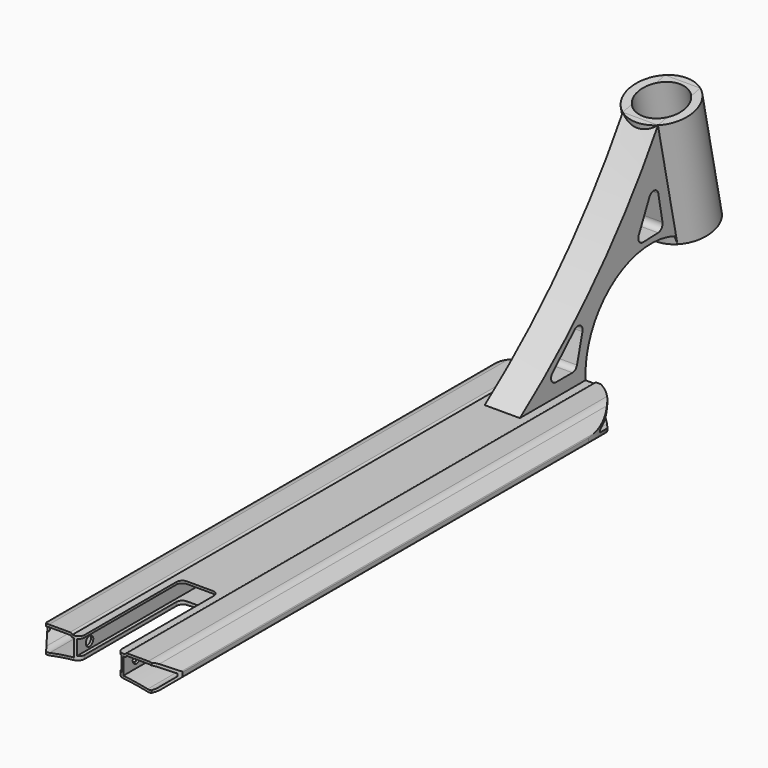
from build123d import *

# Parameters (mm, degrees)
F1_DEPTH       = 250
F2_W           = 38
F2_H           = 13
F3_DEPTH       = 500.001
F4_T1_DEPTH    = 509.3674969976
F5_R           = 9
F6_R           = 1
F8_DEPTH       = 500.001
F10_DEPTH      = 21.9508968951
F10_DEPTH_BACK = 1.301
F12_DEPTH      = 21.9508969951
F12_DEPTH_BACK = 1.3010001
F13_T1_DEPTH   = 2
F13_T6_DEPTH   = 15.5773592081
F13_S7_R       = 200
F13_T8_DEPTH   = 10
F13_T12_DEPTH  = 15.5773592081
F13_S13_R      = 200
F13_T14_DEPTH  = 10
F13_T15_DEPTH  = 28.0773592081
F13_T17_DEPTH  = 27
F15_DEPTH      = 15
F16_R          = 27.5
F17_DEPTH      = 100
F19_D          = 40
F21_D          = 8
F21_DEPTH      = 78.5010001
F23_DEPTH      = 72.5010001
F24_R          = 5


# Not quite as in the source:
# - a fillet or chamfer that OpenCascade refuses, or shapes differently, is made with other operations: its cross-section is extruded or revolved along the edge and cut away or added


with BuildPart() as f1:
    # F0 (on Front) → F1 (new body, symmetric)
    with BuildSketch(Plane.XZ):
        with BuildLine():
            Line((22.5, 0), (0, 0))
            Line((0, 0), (-22.5, 0))
            Line((-22.5, 0), (-22.5, 1.3))
            Line((-22.5, 1.3), (-45.5824640741, 1.3))
            Line((-45.5824640741, 1.3), (-57.5, -8.7))
            Line((-57.5, -8.7), (-57.5, -12.7))
            Line((-57.5, -12.7), (-45.5824640741, -22.7))
            ThreePointArc((-45.5824640741, -22.7), (0, -17.4363319182), (45.5824640741, -22.7))
            Line((45.5824640741, -22.7), (57.5, -12.7))
            Line((57.5, -12.7), (57.5, -8.7))
            Line((57.5, -8.7), (45.5824640741, 1.3))
            Line((45.5824640741, 1.3), (22.5, 1.3))
            Line((22.5, 1.3), (22.5, 0))
        make_face()
    extrude(amount=F1_DEPTH, both=True)

    # F2 (on face) → F3 (cut, through all)
    with BuildSketch(Plane.XZ.offset(250)):
        with Locations((0, -8.5)):
            Rectangle(F2_W, F2_H)
    extrude(amount=-F3_DEPTH, mode=Mode.SUBTRACT)

    # F4: fillet of radius 2 on 2 edges, made by hand

    # F4_s2 → F4_t1 (cut)
    with BuildSketch(Plane.XZ.offset(-254.6837484988)):
        with BuildLine():
            ThreePointArc((-24.3734993995, 1.3), (-23.2333239744, 0.9431676725), (-22.5, 0))
            Line((-22.5, 0), (-22.5, 1.3))
            Line((-22.5, 1.3), (-24.3734993995, 1.3))
        make_face()
        with BuildLine():
            ThreePointArc((24.3734993995, 1.3), (23.2333239744, 0.9431676725), (22.5, 0))
            Line((22.5, 0), (22.5, 1.3))
            Line((22.5, 1.3), (24.3734993995, 1.3))
        make_face()
    extrude(amount=F4_T1_DEPTH, mode=Mode.SUBTRACT)

    # F5
    f5_edges = [f1.edges().sort_by_distance(p)[0] for p in [
        (-45.582464, 0, 1.3),
        (45.582464, 0, 1.3),
        (45.582464, 0, -22.7),
        (-45.582464, 0, -22.7),
    ]]
    fillet(f5_edges, radius=F5_R)

    # F6
    f6_edges = [f1.edges().sort_by_distance(p)[0] for p in [
        (57.5, 0, -8.7),
        (57.5, 0, -12.7),
        (-57.5, 0, -8.7),
        (-57.5, 0, -12.7),
    ]]
    fillet(f6_edges, radius=F6_R)

    # F7 (on face) → F8 (cut, through all)
    with BuildSketch(Plane.XZ.offset(250)):
        with BuildLine():
            ThreePointArc((-41.7537576423, -19.7987248623), (-31.4193924923, -17.8948029689), (-21, -16.5308815192))
            Line((-21, -16.5308815192), (-21, -2))
            Line((-21, -2), (-22.8755325079, -2))
            ThreePointArc((-22.8755325079, -2), (-23.3817957129, -1.070317781), (-24.3734993995, -0.7))
            Line((-24.3734993995, -0.7), (-42.3067319657, -0.7))
            ThreePointArc((-42.3067319657, -0.7), (-44.7008729689, -1.1221516545), (-46.8062452335, -2.3376888982))
            Line((-46.8062452335, -2.3376888982), (-55.5, -9.6326153163))
            Line((-55.5, -9.6326153163), (-55.5, -11.7673846837))
            Line((-55.5, -11.7673846837), (-47.7001833036, -18.3122079969))
            ThreePointArc((-47.7001833036, -18.3122079969), (-44.8983231577, -19.7409184587), (-41.7537576423, -19.7987248623))
        make_face()
        with BuildLine():
            Line((21, -2), (21, -16.5308815192))
            ThreePointArc((21, -16.5308815192), (31.4193924923, -17.8948029689), (41.7537576423, -19.7987248623))
            ThreePointArc((41.7537576423, -19.7987248623), (44.8983231577, -19.7409184587), (47.7001833036, -18.3122079969))
            Line((47.7001833036, -18.3122079969), (55.5, -11.7673846837))
            Line((55.5, -11.7673846837), (55.5, -9.6326153163))
            Line((55.5, -9.6326153163), (46.8062452335, -2.3376888982))
            ThreePointArc((46.8062452335, -2.3376888982), (44.7008729689, -1.1221516545), (42.3067319657, -0.7))
            Line((42.3067319657, -0.7), (24.3734993995, -0.7))
            ThreePointArc((24.3734993995, -0.7), (23.3817957129, -1.070317781), (22.8755325079, -2))
            Line((22.8755325079, -2), (21, -2))
        make_face()
    extrude(amount=-F8_DEPTH, mode=Mode.SUBTRACT)

    # F9 (on Top) → F10 (cut, two sides)
    with BuildSketch(Plane.XY) as f10_sk:
        with BuildLine():
            ThreePointArc((-57.5, 200), (0, 257.5), (57.5, 200))
            Line((57.5, 200), (57.5, 280))
            Line((57.5, 280), (-57.5, 280))
            Line((-57.5, 280), (-57.5, 200))
        make_face()
    extrude(amount=-F10_DEPTH, mode=Mode.SUBTRACT)
    extrude(f10_sk.sketch, amount=F10_DEPTH_BACK, mode=Mode.SUBTRACT)

    # F11 (on Top) → F12 (cut, two sides)
    with BuildSketch(Plane.XY) as f12_sk:
        Polygon((-16, -142.1357727465), (-16, -252.1357727465), (-43.2975540478, -252.1357727465), (-68, -218.1357727465), (-68, -325.6394559335), (0, -325.6394559335), (0, -142.1357727465), align=None)
        Polygon((16, -142.1357727465), (0, -142.1357727465), (0, -325.6394559335), (68, -325.6394559335), (68, -218.1357727465), (43.2975540478, -252.1357727465), (16, -252.1357727465), align=None)
    extrude(amount=-F12_DEPTH, mode=Mode.SUBTRACT)
    extrude(f12_sk.sketch, amount=F12_DEPTH_BACK, mode=Mode.SUBTRACT)

    # F13: fillet of radius 5 on 8 edges, made by hand

    # F13_s2 → F13_t1 (join)
    with BuildSketch(Plane.XY.offset(-2)):
        with BuildLine():
            ThreePointArc((16, -147.1357727465), (14.5355339059, -143.6002388406), (11, -142.1357727465))
            Line((11, -142.1357727465), (16, -142.1357727465))
            Line((16, -142.1357727465), (16, -147.1357727465))
        make_face()
        with BuildLine():
            ThreePointArc((-16, -147.1357727465), (-14.5355339059, -143.6002388406), (-11, -142.1357727465))
            Line((-11, -142.1357727465), (-16, -142.1357727465))
            Line((-16, -142.1357727465), (-16, -147.1357727465))
        make_face()
    extrude(amount=F13_T1_DEPTH)


with BuildPart() as f13_tool4:
    # F13_s5 → F13_t6 (new body)
    with BuildSketch(Plane.XY.offset(-15)):
        with BuildLine():
            ThreePointArc((-16, -147.1357727465), (-14.5355339059, -143.6002388406), (-11, -142.1357727465))
            Line((-11, -142.1357727465), (-16, -142.1357727465))
            Line((-16, -142.1357727465), (-16, -147.1357727465))
        make_face()
    extrude(amount=-F13_T6_DEPTH)

    # F13_s7 → F13_t8 (cut, symmetric)
    with BuildSketch(Plane.XZ.offset(144.6)):
        with Locations((0, -217.4363319182)):
            Circle(F13_S7_R)
    extrude(amount=F13_T8_DEPTH, both=True, mode=Mode.SUBTRACT)


with BuildPart() as f1_1:
    add(f1.part)

    # F13_t3: union F13_tool4
    add(f13_tool4.part)


with BuildPart() as f13_tool10:
    # F13_s11 → F13_t12 (new body)
    with BuildSketch(Plane.XY.offset(-15)):
        with BuildLine():
            ThreePointArc((11, -142.1357727465), (14.5355339059, -143.6002388406), (16, -147.1357727465))
            Line((16, -147.1357727465), (16, -142.1357727465))
            Line((16, -142.1357727465), (11, -142.1357727465))
        make_face()
    extrude(amount=-F13_T12_DEPTH)

    # F13_s13 → F13_t14 (cut, symmetric)
    with BuildSketch(Plane.XZ.offset(144.6)):
        with Locations((0, -217.4363319182)):
            Circle(F13_S13_R)
    extrude(amount=F13_T14_DEPTH, both=True, mode=Mode.SUBTRACT)


with BuildPart() as f1_2:
    add(f1_1.part)

    # F13_t9: union F13_tool10
    add(f13_tool10.part)

    # F13_s16 → F13_t15 (cut)
    with BuildSketch(Plane.XY.offset(-30.5773592081)):
        with BuildLine():
            ThreePointArc((-21, -250), (-17.4644660941, -248.5355339059), (-16, -245))
            Line((-16, -245), (-16, -250))
            Line((-16, -250), (-21, -250))
        make_face()
        with BuildLine():
            ThreePointArc((21, -250), (17.4644660941, -248.5355339059), (16, -245))
            Line((16, -245), (16, -250))
            Line((16, -250), (21, -250))
        make_face()
    extrude(amount=F13_T15_DEPTH, mode=Mode.SUBTRACT)

    # F13_s18 → F13_t17 (cut)
    with BuildSketch(Plane.XY.offset(-14.5)):
        with BuildLine():
            ThreePointArc((21, -250), (17.4644660941, -248.5355339059), (16, -245))
            Line((16, -245), (16, -250))
            Line((16, -250), (21, -250))
        make_face()
        with BuildLine():
            ThreePointArc((-21, -250), (-17.4644660941, -248.5355339059), (-16, -245))
            Line((-16, -245), (-16, -250))
            Line((-16, -250), (-21, -250))
        make_face()
    extrude(amount=F13_T17_DEPTH, mode=Mode.SUBTRACT)

    # F14 (on Right) → F15 (join, symmetric)
    with BuildSketch(Plane.YZ):
        with BuildLine():
            Line((180.1167654991, 0), (250.1167654991, 0))
            ThreePointArc((250.1167654991, 0), (278.9952668686, 60.8945120165), (345.877289772, 69.195382297))
            Line((345.877289772, 69.195382297), (348.1046356057, 62.1916612076))
            Line((348.1046356057, 62.1916612076), (393.0964714503, 71.7694849343))
            Line((393.0964714503, 71.7694849343), (372.2751155226, 169.5778237267))
            Line((372.2751155226, 169.5778237267), (327.2832796781, 160))
            ThreePointArc((327.2832796781, 160), (261.6838080328, 72.6565882889), (180.1167654991, 0))
        make_face()
    extrude(amount=F15_DEPTH, both=True)

    # F16 (on face) → F17 (join, through all)
    with BuildSketch(Plane(origin=(0, -18.3953609542, 86.4122251533), x_dir=(1, 0, 0), z_dir=(0, -0.2082135593, 0.9780833879))):
        with Locations((0, 376.4245084828)):
            Circle(F16_R)
    extrude(amount=-F17_DEPTH)

    # F19 (through all)
    with Locations(Plane(origin=(0, -18.3953609542, 86.4122251533), x_dir=(1, 0, 0), z_dir=(0, -0.2082135593, 0.9780833879))):
        with Locations((0, 376.4245084828)):
            Hole(F19_D / 2)

    # F21 (through all, one way)
    with BuildSketch(Plane.YZ.offset(21)):
        with Locations((-236, -9.2654407596)):
            Circle(F21_D / 2)
    extrude(amount=-F21_DEPTH, mode=Mode.SUBTRACT)

    # F22 (on face) → F23 (cut, through all)
    with BuildSketch(Plane.YZ.offset(15)):
        Polygon((251.1910329444, 54.8862453262), (206, 11.3), (240, 11.3), align=None)
        Polygon((324.7441051812, 123.6654943361), (303.2328515089, 78.2494083459), (333.2080655824, 79.4686463226), align=None)
    extrude(amount=-F23_DEPTH, mode=Mode.SUBTRACT)

    # F24
    f24_edges = [f1_2.edges().sort_by_distance(p)[0] for p in [
        (0, 206, 11.3),
        (0, 240, 11.3),
        (0, 251.191033, 54.886245),
        (0, 324.744105, 123.665494),
        (0, 303.232852, 78.249408),
        (0, 333.208066, 79.468646),
    ]]
    fillet(f24_edges, radius=F24_R)


solid = f1_2.part
